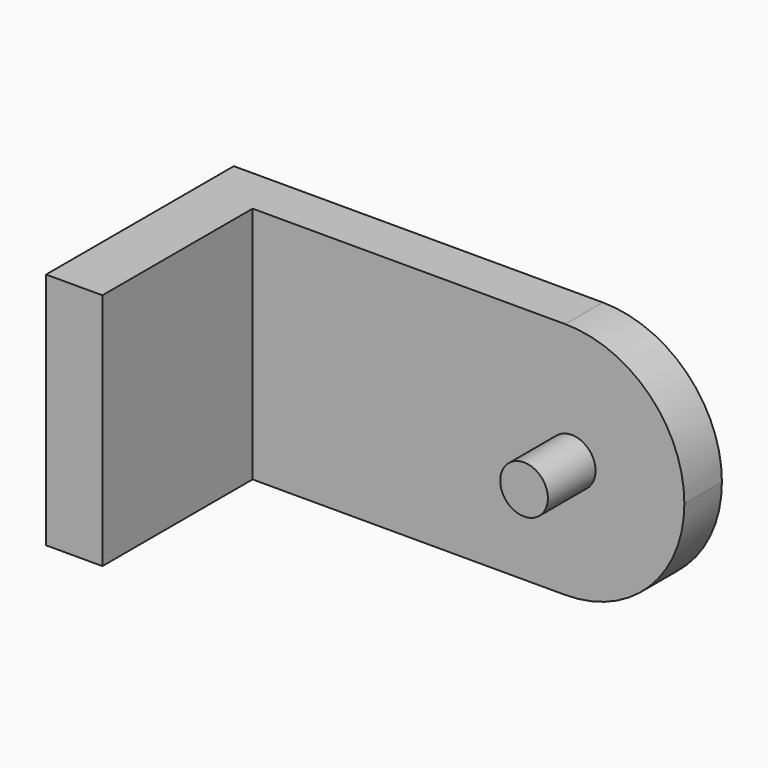
from build123d import *

# Parameters (mm, degrees)
F1_DEPTH = 12.7
F2_R     = 1.27
F3_DEPTH = 3.175
F4_R     = 6.34999


# Not quite as in the source:
# - a fillet or chamfer is up to 0.001 mm smaller than in the source, because OpenCascade refuses the exact size


with BuildPart() as f1:
    # F0 (on Top) → F1 (new body)
    with BuildSketch(Plane.XY):
        Polygon((0, -12.5), (3, -12.5), (3, -2.5), (26, -2.5), (26, 0), (0, 0), align=None)
    extrude(amount=F1_DEPTH)

    # F2 (on face) → F3 (join)
    with BuildSketch(Plane.XZ.offset(2.5)):
        with Locations((20, 6.35)):
            Circle(F2_R)
    extrude(amount=F3_DEPTH)

    # F4 (radius 6.35 in the source; OpenCascade refuses exactly that, so slightly less here)
    f4_edges = [f1.edges().sort_by_distance(p)[0] for p in [
        (26, -1.25, 12.7),
        (26, -1.25, 0),
    ]]
    fillet(f4_edges, radius=F4_R)


solid = f1.part
